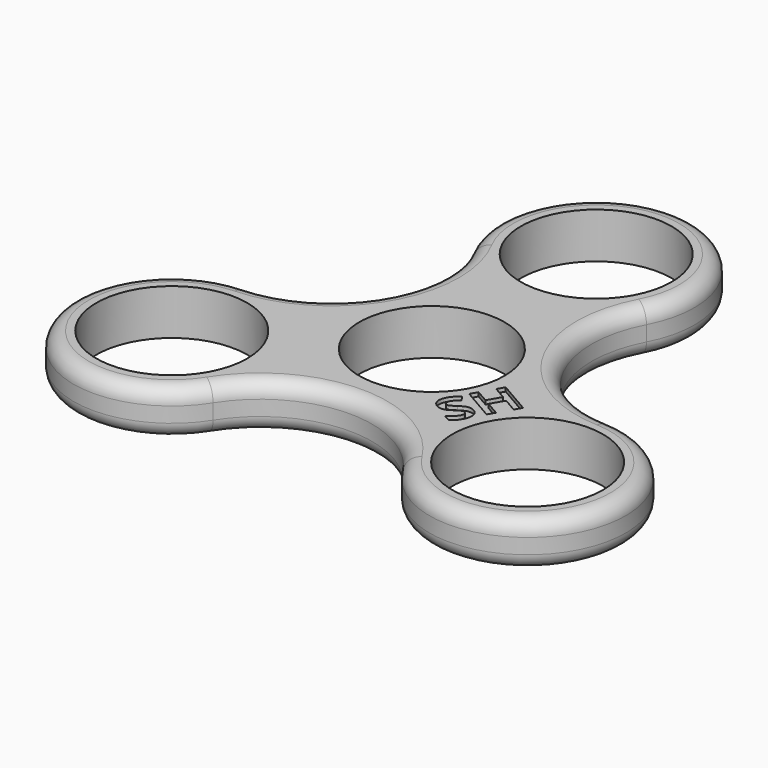
from build123d import *

# Parameters (mm, degrees)
F0_R         = 9.91
F0_R_2       = 9.55
F1_DEPTH     = 6
F2_R         = 2
F3_TEXT_SIZE = 6.8784320588
F4_DEPTH     = 0.5


# Not quite as in the source:
# - Text() gives the source's letters only with a copy of the font that has no kerning and outlines rounded to 1/6400 em; it was checked with that copy


with BuildPart() as f1:
    # F0 (on Top) → F1 (new body)
    with BuildSketch(Plane.XY):
        with BuildLine():
            ThreePointArc((23.8765271258, -0.5994488162), (11.6913429511, 6.75), (11.4191256598, 20.9774034532))
            ThreePointArc((11.4191256598, 20.9774034532), (0, 39.91), (-11.4191256598, 20.9774034532))
            ThreePointArc((-11.4191256598, 20.9774034532), (-11.6913429511, 6.75), (-23.8765271258, -0.5994488162))
            ThreePointArc((-23.8765271258, -0.5994488162), (-34.563073865, -19.955), (-12.457401466, -20.377954637))
            ThreePointArc((-12.457401466, -20.377954637), (0, -13.5), (12.457401466, -20.377954637))
            ThreePointArc((12.457401466, -20.377954637), (34.563073865, -19.955), (23.8765271258, -0.5994488162))
        make_face()
        with Locations((-23.3826859022, -13.5)):
            Circle(F0_R, mode=Mode.SUBTRACT)
        with Locations((23.3826859022, -13.5)):
            Circle(F0_R, mode=Mode.SUBTRACT)
        Circle(F0_R_2, mode=Mode.SUBTRACT)
        with Locations((0, 27)):
            Circle(F0_R, mode=Mode.SUBTRACT)
    extrude(amount=F1_DEPTH)

    # F2
    f2_edges = [f1.edges().sort_by_distance(p)[0] for p in [
        (0, -13.5, 6),
        (0, -13.5, 0),
    ]]
    fillet(f2_edges, radius=F2_R)

    # F3 (on face) → F4 (cut)
    with BuildSketch(Plane.XY.offset(6)):
        with Locations(Location((11.2719813881, -11.6723955894), (0, 0, 60))):
            Text('SH', F3_TEXT_SIZE, font='Open Sans', font_style=FontStyle.BOLD, text_align=(TextAlign.LEFT, TextAlign.BOTTOM))
    extrude(amount=-F4_DEPTH, mode=Mode.SUBTRACT)


solid = f1.part
